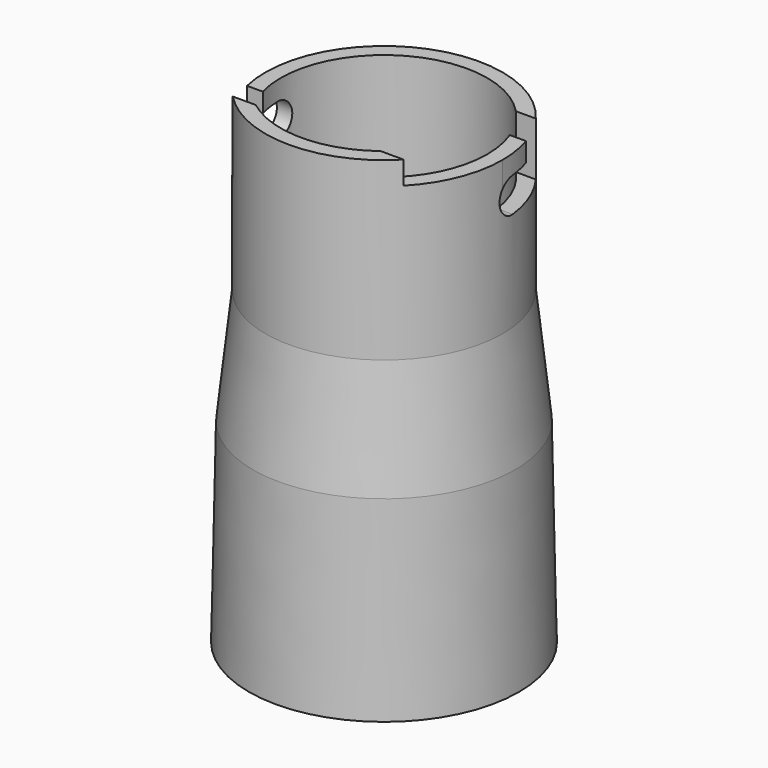
from build123d import *

# Parameters (mm, degrees)
F0_R          = 15.5
F0_R_2        = 13.5
F1_DEPTH      = 23
F2_W          = 26.25
F2_H          = 3
F3_DEPTH      = 62
F3_DEPTH_BACK = 62
F6_REACH      = 29.8275487819
F7_REACH      = 27.5036039842


# Not quite as in the source:
# - an extrude ends at something that could not be found from the text; its depth is read off the source's solid


with BuildPart() as f1:
    # F0 (on Top) → F1 (new body)
    with BuildSketch(Plane.XY):
        Circle(F0_R)
        Circle(F0_R_2, mode=Mode.SUBTRACT)
    extrude(amount=F1_DEPTH)

    # F2 (on Right) → F3 (cut, two sides)
    with BuildSketch(Plane.YZ) as f3_sk:
        with Locations((2.375, 21.5)):
            Rectangle(F2_W, F2_H)
    extrude(amount=-F3_DEPTH, mode=Mode.SUBTRACT)
    extrude(f3_sk.sketch, amount=F3_DEPTH_BACK, mode=Mode.SUBTRACT)

    f6_end = f1.faces().sort_by_distance((-15.5, 0, 11.5))[0]
    # F4 (on Right) → F6 (cut, up to a face of the model that its end follows)
    with BuildSketch(Plane.YZ):
        with BuildLine():
            Line((-3.5, 20), (-10.75, 20))
            Line((-10.75, 20), (-10.75, 13))
            Line((-10.75, 13), (-0.5, 13))
            ThreePointArc((-0.5, 13), (1.75, 15.25), (-0.5, 17.5))
            Line((-0.5, 17.5), (-3.5, 17.5))
            Line((-3.5, 17.5), (-3.5, 20))
        make_face()
    f6_long = extrude(amount=-F6_REACH, mode=Mode.PRIVATE)
    add(split(f6_long, bisect_by=f6_end, keep=Keep.BOTTOM, mode=Mode.PRIVATE), mode=Mode.SUBTRACT)

    f7_end = f1.faces().sort_by_distance((-15.5, 0, 11.5))[0]
    # F5 (on Right) → F7 (cut, up to a face of the model that its end follows)
    with BuildSketch(Plane.YZ):
        with BuildLine():
            Line((4.75, 20), (4.75, 17.5))
            Line((4.75, 17.5), (1.75, 17.5))
            ThreePointArc((1.75, 17.5), (-0.5, 15.25), (1.75, 13))
            Line((1.75, 13), (9.25, 13))
            Line((9.25, 13), (9.25, 20))
            Line((9.25, 20), (4.75, 20))
        make_face()
    f7_long = extrude(amount=F7_REACH, mode=Mode.PRIVATE)
    add(split(f7_long, bisect_by=f7_end, keep=Keep.BOTTOM, mode=Mode.PRIVATE), mode=Mode.SUBTRACT)

    # F10 (on Front) → F11 (revolve)
    with BuildSketch(Plane.XZ):
        Polygon((-15.15, -15.1), (-13.5, 0), (-15.5, 0), (-17.15, -15.1), align=None)
    revolve(axis=Axis((0, 0, -0.5375670735), (0, 0, -1)))

    # F14 (on Front) → F15 (revolve)
    with BuildSketch(Plane.XZ):
        Polygon((-15.15, -15.1), (-17.15, -15.1), (-17.65, -40.5), (-15.65, -40.5), align=None)
    revolve(axis=Axis((0, 0, -27.8), (0, 0, 1)))


solid = f1.part
